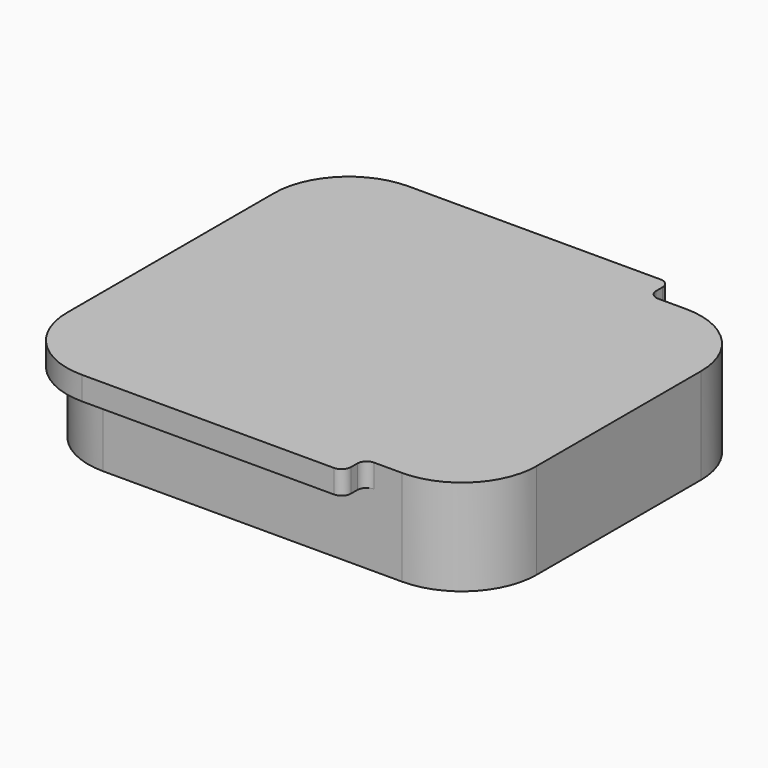
from build123d import *

# Parameters (mm, degrees)
F1_DEPTH     = 10.25
F3_DEPTH     = 2.5
F4_R         = 1
F5_T         = 1.9
F5_T3_DEPTH  = 4.8
F5_T5_DEPTH  = 31.8
F5_T8_ANGLE  = 90.000000001
F5_T10_ANGLE = 90.000000001
F6_R         = 5.5
F7_DEPTH     = 2


# Not quite as in the source:
# - a shell that OpenCascade refuses in one call is made with other operations: the cavity is built on its own and cut out


with BuildPart() as f1:
    # F0 (on Top) → F1 (new body)
    with BuildSketch(Plane.XY):
        with BuildLine():
            Line((16, 19), (-16, 19))
            ThreePointArc((-16, 19), (-21.6568542495, 16.6568542495), (-24, 11))
            Line((-24, 11), (-24, -11))
            ThreePointArc((-24, -11), (-21.6568542495, -16.6568542495), (-16, -19))
            Line((-16, -19), (16, -19))
            ThreePointArc((16, -19), (21.6568542495, -16.6568542495), (24, -11))
            Line((24, -11), (24, 11))
            ThreePointArc((24, 11), (21.6568542495, 16.6568542495), (16, 19))
        make_face()
    extrude(amount=F1_DEPTH)

    # F2 (on face) → F3 (join)
    with BuildSketch(Plane.XY.offset(10.25)):
        with BuildLine():
            Line((12, 21.85), (-16, 21.85))
            ThreePointArc((-16, 21.85), (-21.6568542495, 19.5068542495), (-24, 13.85))
            Line((-24, 13.85), (-24, 11))
            ThreePointArc((-24, 11), (-21.6568542495, 16.6568542495), (-16, 19))
            Line((-16, 19), (12, 19))
            Line((12, 19), (12, 21.85))
        make_face()
        with BuildLine():
            Line((12, -21.85), (12, -19))
            Line((12, -19), (-16, -19))
            ThreePointArc((-16, -19), (-21.6568542495, -16.6568542495), (-24, -11))
            Line((-24, -11), (-24, -13.85))
            ThreePointArc((-24, -13.85), (-21.6568542495, -19.5068542495), (-16, -21.85))
            Line((-16, -21.85), (12, -21.85))
        make_face()
    extrude(amount=-F3_DEPTH)

    # F4
    f4_edges = [f1.edges().sort_by_distance(p)[0] for p in [
        (12, -21.85, 9),
        (12, -19, 9),
        (12, 19, 9),
        (12, 21.85, 9),
    ]]
    fillet(f4_edges, radius=F4_R)

    # F5: shell of thickness 1.9, made by hand


with BuildPart() as f5_core1:
    # F5_t2: copy of F1
    add(f1.part)

    # the walls: a layer under each face that stays
    f5_faces = [f5_core1.faces().sort_by_distance(p)[0] for p in [
        (0, 19, 5.125),
        (0, 0, 10.25),
        (12.2928932188, 19.2928932188, 9),
        (21.6568542495, 16.6568542495, 5.125),
        (-17.8333333333, 20.0416666667, 7.75),
        (-21.6568542495, 16.6568542495, 3.875),
        (12, 20.425, 9),
        (24, 0, 5.125),
        (21.6568542495, -16.6568542495, 5.125),
        (-2.5, 21.85, 9),
        (0, -19, 5.125),
        (-21.6568542495, 19.5068542495, 9),
        (12.2928932188, -19.2928932188, 9),
        (-24, 0, 5.125),
        (12, -20.425, 9),
        (-21.6568542495, -19.5068542495, 9),
        (-2.5, -21.85, 9),
        (-21.6568542495, -16.6568542495, 3.875),
        (-17.8333333333, -20.0416666667, 7.75),
    ]]
    thicken(f5_faces, amount=-F5_T, mode=Mode.SUBTRACT)

    # F5_s4 → F5_t3 (cut)
    with BuildSketch(Plane.YZ.offset(10.1)):
        Polygon((19.019, 7.731), (17.1, 7.75), (17.1, 9.65), (19, 9.65), align=None)
        Polygon((-19.019, 7.731), (-17.1, 7.75), (-17.1, 9.65), (-19, 9.65), align=None)
    extrude(amount=F5_T3_DEPTH, mode=Mode.SUBTRACT)

    # F5_s6 → F5_t5 (cut)
    with BuildSketch(Plane.YZ.offset(-17.9)):
        Polygon((19.019, 7.731), (17.1, 7.75), (17.1, 9.65), (19, 9.65), align=None)
        Polygon((-19.019, 7.731), (-17.1, 7.75), (-17.1, 9.65), (-19, 9.65), align=None)
    extrude(amount=F5_T5_DEPTH, mode=Mode.SUBTRACT)

    # F5_s7 → F5_t8 (revolve, cut)
    with BuildSketch(Plane.XZ.offset(-11)):
        Polygon((-24.019, 7.731), (-24, 9.65), (-22.1, 9.65), (-22.1, 7.75), align=None)
    revolve(axis=Axis((-16, 11, 7.75), (0, 0, -1)), revolution_arc=F5_T8_ANGLE, mode=Mode.SUBTRACT)

    # F5_s9 → F5_t10 (revolve, cut)
    with BuildSketch(Plane.YZ.offset(-16)):
        Polygon((-19.019, 7.731), (-17.1, 7.75), (-17.1, 9.65), (-19, 9.65), align=None)
    revolve(axis=Axis((-16, -11, 7.75), (0, 0, -1)), revolution_arc=F5_T10_ANGLE, mode=Mode.SUBTRACT)


with BuildPart() as f1_1:
    add(f1.part)

    # what is left inside the walls is the cavity
    f5_cavity = [f5_core1.part.solids().sort_by_distance(p)[0] for p in [
        (0, -5.7, 8.331),
    ]]
    add(f5_cavity, mode=Mode.SUBTRACT)

    # F6 (on face) → F7 (cut)
    with BuildSketch(Plane(origin=(-24, 0, 0), x_dir=(0, -1, 0), z_dir=(-1, 0, 0))):
        Circle(F6_R)
    extrude(amount=-F7_DEPTH, mode=Mode.SUBTRACT)


solid = f1_1.part
